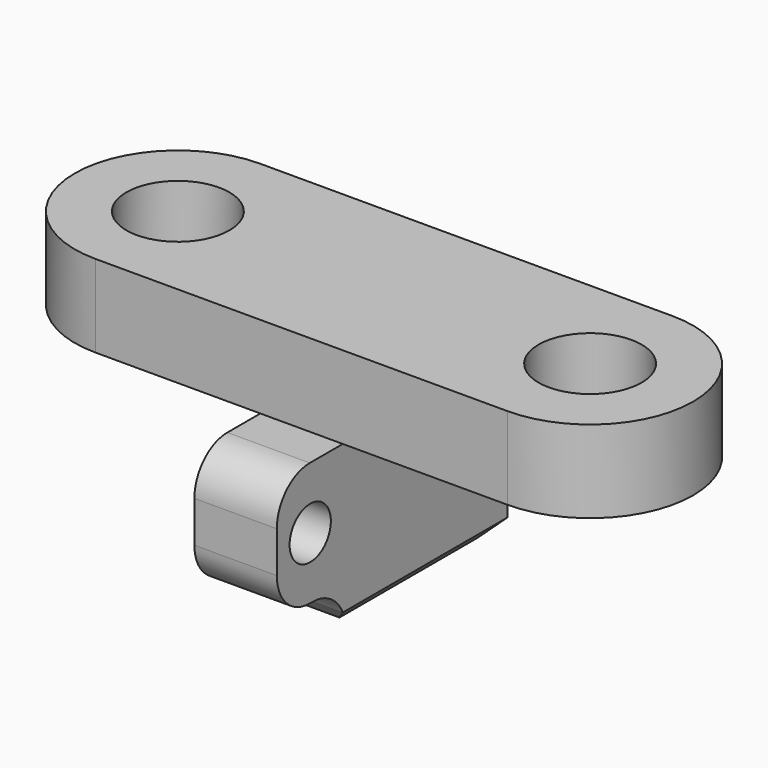
from build123d import *

# Parameters (mm, degrees)
F0_R         = 3.175
F1_DEPTH     = 22.86
F2_W         = 6.35
F2_H         = 6.35
F2_W_2       = 6.7925655007
F3_DEPTH     = 25.4
F5_DEPTH     = 25.4
F6_SIZE      = 1.016
F7_W         = 5.08
F7_H         = 7.62
F8_DEPTH     = 5.08
F9_R         = 1.5875
F10_DEPTH    = 25.4
F11_T1_DEPTH = 5.08
F11_T3_DEPTH = 17.78
F11_T5_DEPTH = 17.78


# Not quite as in the source:
# - a fillet or chamfer that OpenCascade refuses, or shapes differently, is made with other operations: its cross-section is extruded or revolved along the edge and cut away or added


with BuildPart() as f1:
    # F0 (on Top) → F1 (new body)
    with BuildSketch(Plane.XY):
        with BuildLine():
            Line((0, 6.35), (-25.4, 6.35))
            ThreePointArc((-25.4, 6.35), (-31.75, 0), (-25.4, -6.35))
            Line((-25.4, -6.35), (0, -6.35))
            ThreePointArc((0, -6.35), (6.35, 0), (0, 6.35))
        make_face()
        with Locations((-25.4, 0)):
            Circle(F0_R, mode=Mode.SUBTRACT)
        with BuildLine():
            ThreePointArc((3.175, 0), (0, -3.175), (-3.175, 0))
            ThreePointArc((-3.175, 0), (0, 3.175), (3.175, 0))
        make_face(mode=Mode.SUBTRACT)
    extrude(amount=F1_DEPTH)

    # F2 (on face) → F3 (cut)
    with BuildSketch(Plane(origin=(0, 6.35, 0), x_dir=(-1, 0, 0), z_dir=(0, 1, 0))):
        with Locations((-3.175, 8.255)):
            Rectangle(F2_W, F2_H)
        with Locations((28.7962827504, 14.605)):
            Rectangle(F2_W_2, F2_H)
        with Locations((28.7962827504, 8.255)):
            Rectangle(F2_W_2, F2_H)
        with Locations((3.175, 8.255)):
            Rectangle(F2_W, F2_H)
        with Locations((3.175, 14.605)):
            Rectangle(F2_W, F2_H)
        with Locations((22.225, 14.605)):
            Rectangle(F2_W, F2_H)
        with Locations((22.225, 8.255)):
            Rectangle(F2_W, F2_H)
        with Locations((-3.175, 14.605)):
            Rectangle(F2_W, F2_H)
    extrude(amount=-F3_DEPTH, mode=Mode.SUBTRACT)

    # F4 (on face) → F5 (cut)
    with BuildSketch(Plane(origin=(0, 6.35, 0), x_dir=(-1, 0, 0), z_dir=(0, 1, 0))):
        Polygon((10.16, 17.78), (6.35, 17.78), (-14.3396928906, 11.8959285319), (-15.9743130207, -5.6489794515), (34.4809181988, -5.6489794515), (40.5834950507, 3.3959113061), (19.05, 17.78), (15.24, 17.78), (15.24, 7.62), (10.16, 7.62), align=None)
    extrude(amount=-F5_DEPTH, mode=Mode.SUBTRACT)

    # F6
    f6_edges = [f1.edges().sort_by_distance(p)[0] for p in [
        (-15.24, 0, 7.62),
        (-10.16, 0, 7.62),
        (-12.7, -6.35, 7.62),
        (-12.7, 6.35, 7.62),
    ]]
    chamfer(f6_edges, length=F6_SIZE)

    # F7 (on face) → F8 (join)
    with BuildSketch(Plane.XZ.offset(6.35)):
        with Locations((-12.7, 13.97)):
            Rectangle(F7_W, F7_H)
    extrude(amount=F8_DEPTH)

    # F9 (on face) → F10 (cut)
    with BuildSketch(Plane(origin=(-15.24, 0, 0), x_dir=(0, -1, 0), z_dir=(-1, 0, 0))):
        with Locations((8.8569838554, 13.97)):
            Circle(F9_R)
    extrude(amount=-F10_DEPTH, mode=Mode.SUBTRACT)

    # F11: fillet of radius 2.54 on 3 edges, made by hand

    # F11_s2 → F11_t1 (join)
    with BuildSketch(Plane.YZ.offset(-15.24)):
        with BuildLine():
            ThreePointArc((-8.677948453, 10.16), (-7.286733157, 9.7451164674), (-6.35, 8.636))
            Line((-6.35, 8.636), (-6.35, 10.16))
            Line((-6.35, 10.16), (-8.677948453, 10.16))
        make_face()
    extrude(amount=F11_T1_DEPTH)

    # F11_s4 → F11_t3 (cut)
    with BuildSketch(Plane.YZ.offset(-21.59)):
        with BuildLine():
            ThreePointArc((-8.89, 17.78), (-10.6860512242, 17.0360512242), (-11.43, 15.24))
            Line((-11.43, 15.24), (-11.43, 17.78))
            Line((-11.43, 17.78), (-8.89, 17.78))
        make_face()
    extrude(amount=F11_T3_DEPTH, mode=Mode.SUBTRACT)

    # F11_s6 → F11_t5 (cut)
    with BuildSketch(Plane.YZ.offset(-21.59)):
        with BuildLine():
            ThreePointArc((-8.89, 10.16), (-10.6860512242, 10.9039487758), (-11.43, 12.7))
            Line((-11.43, 12.7), (-11.43, 10.16))
            Line((-11.43, 10.16), (-8.89, 10.16))
        make_face()
    extrude(amount=F11_T5_DEPTH, mode=Mode.SUBTRACT)


solid = f1.part
